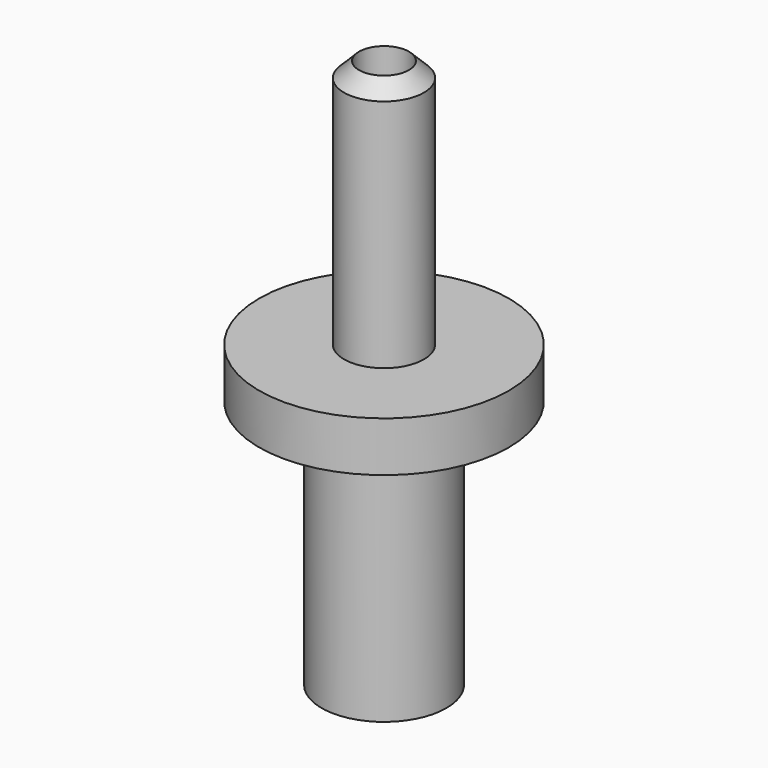
from build123d import *

# Parameters (mm, degrees)
F2_SIZE = 0.76199


# Not quite as in the source:
# - a fillet or chamfer is up to 0.001 mm smaller than in the source, because OpenCascade refuses the exact size


with BuildPart() as f1:
    # F0 (on Front) → F1 (revolve)
    with BuildSketch(Plane.XZ):
        Polygon((2.032, 0), (1.27, 0), (1.27, -13.97), (1.27, -27.94), (3.175, -27.94), (3.175, -15.24), (6.35, -15.24), (6.35, -12.7), (2.032, -12.7), align=None)
    revolve(axis=Axis((0, 0, -18.8239812851), (0, 0, -1)))

    # F2 (size 0.762 in the source; OpenCascade refuses exactly that, so slightly less here)
    f2_edges = [f1.edges().sort_by_distance(p)[0] for p in [
        (-2.032, 0, 0),
    ]]
    chamfer(f2_edges, length=F2_SIZE)


solid = f1.part
